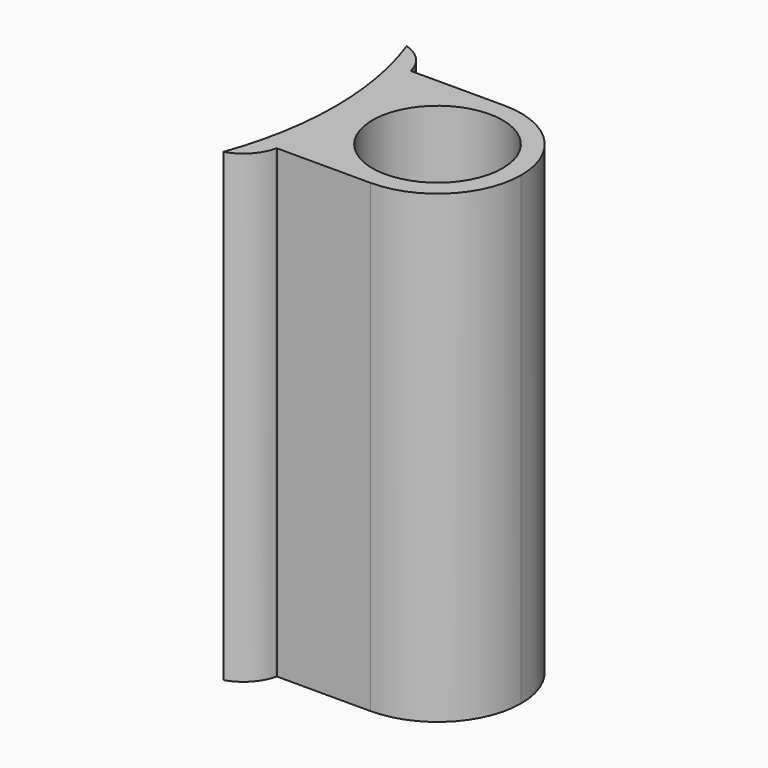
from build123d import *

# Parameters (mm, degrees)
F0_R        = 3.5
F1_DEPTH    = 25
F2_T1_DEPTH = 35.23561564
F2_T3_DEPTH = 35.4401476299


# Not quite as in the source:
# - a fillet or chamfer that OpenCascade refuses, or shapes differently, is made with other operations: its cross-section is extruded or revolved along the edge and cut away or added


with BuildPart() as f1:
    # F0 (on Top) → F1 (new body)
    with BuildSketch(Plane.XY):
        with BuildLine():
            ThreePointArc((23.5, 4.5), (20.3180194847, 3.1819805153), (19, 0))
            ThreePointArc((19, 0), (20.3180194847, -3.1819805153), (23.5, -4.5))
            ThreePointArc((23.5, -4.5), (26.6819805153, -3.1819805153), (28, 0))
            ThreePointArc((28, 0), (26.6819805153, 3.1819805153), (23.5, 4.5))
        make_face()
        with Locations((23.5, 0)):
            Circle(F0_R, mode=Mode.SUBTRACT)
        with BuildLine():
            ThreePointArc((18.459414942, 4.5), (18.8643696409, 2.2661769682), (19, 0))
            ThreePointArc((19, 0), (20.3180194847, 3.1819805153), (23.5, 4.5))
            Line((23.5, 4.5), (18.459414942, 4.5))
        make_face()
        with BuildLine():
            ThreePointArc((23.5, -4.5), (20.3180194847, -3.1819805153), (19, 0))
            ThreePointArc((19, 0), (18.8643696409, -2.2661769682), (18.459414942, -4.5))
            Line((18.459414942, -4.5), (23.5, -4.5))
        make_face()
        with BuildLine():
            ThreePointArc((18.459414942, -4.5), (18.8643696409, -2.2661769682), (19, 0))
            ThreePointArc((19, 0), (18.8643696409, 2.2661769682), (18.459414942, 4.5))
            ThreePointArc((18.459414942, 4.5), (18.1842599773, 5.507512059), (17.8541597949, 6.4983827232))
            Line((17.8541597949, 6.4983827232), (16.9144671741, 6.1563625799))
            ThreePointArc((16.9144671741, 6.1563625799), (17.7265395542, 3.125667198), (18, 0))
            ThreePointArc((18, 0), (17.7265395542, -3.125667198), (16.9144671741, -6.1563625799))
            Line((16.9144671741, -6.1563625799), (17.8541597949, -6.4983827232))
            ThreePointArc((17.8541597949, -6.4983827232), (18.1842599773, -5.507512059), (18.459414942, -4.5))
        make_face()
    extrude(amount=F1_DEPTH)

    # F2: fillet of radius 2.25 on 2 edges, made by hand

    # F2_s2 → F2_t1 (cut)
    with BuildSketch(Plane.XY.offset(-5.11780782)):
        with BuildLine():
            ThreePointArc((16.9144671741, -6.1563625799), (17.8963613222, -5.5515835221), (18.4496693096, -4.5397910048))
            Line((18.4496693096, -4.5397910048), (18.4933658948, -4.5505431414))
            ThreePointArc((18.4933658948, -4.5505431414), (18.2213657624, -5.5402034939), (17.8964459629, -6.5137736296))
            Line((17.8964459629, -6.5137736296), (17.8387688885, -6.5406688911))
            ThreePointArc((17.8387688885, -6.5406688911), (17.3689225781, -6.3696588195), (16.9274597166, -6.1994461479))
            Line((16.9274597166, -6.1994461479), (16.9144671741, -6.1563625799))
        make_face()
    extrude(amount=F2_T1_DEPTH, mode=Mode.SUBTRACT)

    # F2_s4 → F2_t3 (cut)
    with BuildSketch(Plane.XY.offset(-5.2200738149)):
        with BuildLine():
            ThreePointArc((18.459414942, 4.5), (17.9105670548, 5.5367651403), (16.9144671741, 6.1563625799))
            Line((16.9144671741, 6.1563625799), (16.9274524792, 6.1994483299))
            ThreePointArc((16.9274524792, 6.1994483299), (17.3689225781, 6.3696588195), (17.8387688885, 6.5406688911))
            Line((17.8387688885, 6.5406688911), (17.8964459629, 6.5137736296))
            ThreePointArc((17.8964459629, 6.5137736296), (18.2273279614, 5.5205561665), (18.5032992024, 4.5099584984))
            Line((18.5032992024, 4.5099584984), (18.459414942, 4.5))
        make_face()
    extrude(amount=F2_T3_DEPTH, mode=Mode.SUBTRACT)


solid = f1.part
